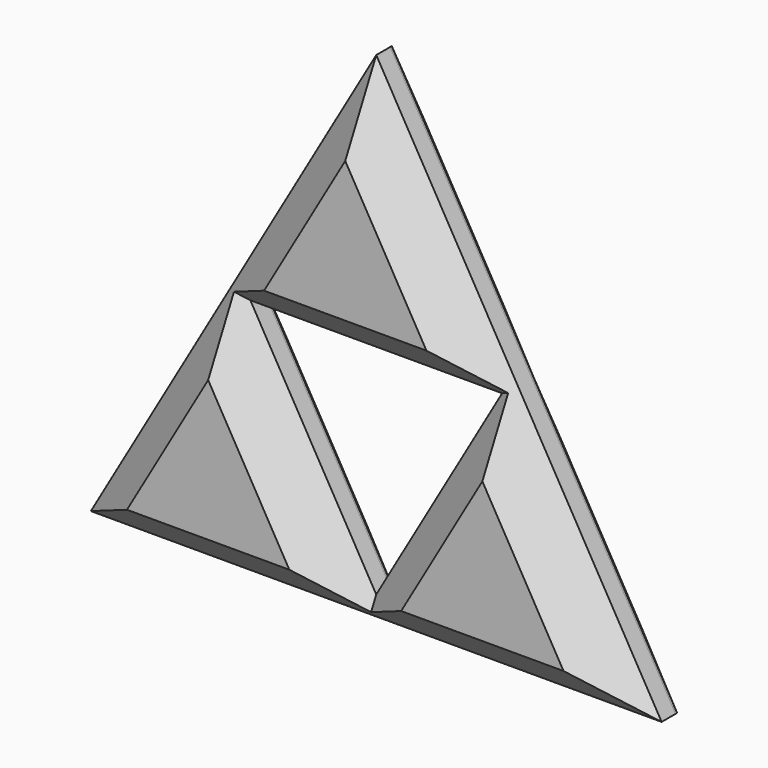
from build123d import *

# Parameters (mm, degrees)
F1_DEPTH      = 12.7
F2_T1_DEPTH   = 100.9671172602
F2_T3_DEPTH   = 100.9671172602
F2_T5_DEPTH   = 100.9671172602
F2_T10_DEPTH  = 59.1482991577
F2_T16_DEPTH  = 59.1482991577
F2_T22_DEPTH  = 59.1482991577
F2_T28_DEPTH  = 59.1482991577
F2_T34_DEPTH  = 59.1482991577
F2_T40_DEPTH  = 59.1482991577
F2_T47_DEPTH  = 59.1482991577
F2_T52_DEPTH  = 59.1482991577
F2_T60_DEPTH  = 59.1482991577
F2_T65_DEPTH  = 59.1482991577
F2_T73_DEPTH  = 59.1482991577
F2_T78_DEPTH  = 59.1482991577
F2_T86_DEPTH  = 59.1482991577
F2_T91_DEPTH  = 59.1482991577
F2_T99_DEPTH  = 59.1482991577
F2_T104_DEPTH = 59.1482991577
F2_T112_DEPTH = 59.1482991577
F2_T117_DEPTH = 59.1482991577
F3_DEPTH      = 2.286
F4_DEPTH      = 2.286


# Not quite as in the source:
# - a fillet or chamfer that OpenCascade refuses, or shapes differently, is made with other operations: its cross-section is extruded or revolved along the edge and cut away or added


with BuildPart() as f1:
    # F0 (on Front) → F1 (new body)
    with BuildSketch(Plane.XZ):
        Polygon((0, 57.1923176659), (-16.51, 28.596158833), (16.51, 28.596158833), align=None)
        Polygon((-33.02, 0), (0, 0), (-16.51, 28.596158833), align=None)
        Polygon((16.51, 28.596158833), (0, 0), (33.02, 0), align=None)
        Polygon((-37.4194090512, -2.54), (-33.02, 0), (-16.51, 28.596158833), (0, 57.1923176659), (0, 62.2723176659), align=None)
        Polygon((16.51, 28.596158833), (33.02, 0), (37.4194090512, -2.54), (0, 62.2723176659), (0, 57.1923176659), align=None)
        Polygon((33.02, 0), (0, 0), (-33.02, 0), (-37.4194090512, -2.54), (37.4194090512, -2.54), align=None)
    extrude(amount=F1_DEPTH)

    # F2: chamfer of 5.08 on 12 edges, made by hand

    # F2_s2 → F2_t1 (cut)
    with BuildSketch(Plane(origin=(33.496779315, 0, 58.0181236636), x_dir=(0, 1, 0), z_dir=(-0.5, 0, -0.8660254038))):
        Polygon((-7.62, -31.136158833), (-12.7, -26.056158833), (-12.7, -31.136158833), align=None)
        Polygon((-5.08, -31.136158833), (0, -26.056158833), (0, -31.136158833), align=None)
    extrude(amount=F2_T1_DEPTH, mode=Mode.SUBTRACT)

    # F2_s4 → F2_t3 (cut)
    with BuildSketch(Plane(origin=(16.986779315, 0, -29.4219648306), x_dir=(0, 1, 0), z_dir=(-0.5, 0, 0.8660254038))):
        Polygon((-7.62, -31.136158833), (-12.7, -26.056158833), (-12.7, -31.136158833), align=None)
        Polygon((-5.08, -31.136158833), (0, -26.056158833), (0, -31.136158833), align=None)
    extrude(amount=F2_T3_DEPTH, mode=Mode.SUBTRACT)

    # F2_s6 → F2_t5 (cut)
    with BuildSketch(Plane.YZ.offset(-50.4835586301)):
        Polygon((-7.62, -2.54), (-12.7, 2.54), (-12.7, -2.54), align=None)
        Polygon((-5.08, -2.54), (0, 2.54), (0, -2.54), align=None)
    extrude(amount=F2_T5_DEPTH, mode=Mode.SUBTRACT)


with BuildPart() as f2_tool8:
    # F2_s9 → F2_t10 (new body)
    with BuildSketch(Plane(origin=(6.5320747894, 0, -11.3138854141), x_dir=(0, 1, 0), z_dir=(-0.5, 0, 0.8660254038))):
        Polygon((-7.62, 0), (-12.7, 5.08), (-12.7, 0), align=None)
    extrude(amount=F2_T10_DEPTH)

    split(bisect_by=Plane(origin=(0, 0, 0), x_dir=(0, 1, 0), z_dir=(-0.8660254038, 0, 0.5)), keep=Keep.TOP)

    split(bisect_by=Plane.XY.offset(28.596158833), keep=Keep.BOTTOM)


with BuildPart() as f1_1:
    add(f1.part)

    # F2_t7: cut F2_tool8
    add(f2_tool8.part, mode=Mode.SUBTRACT)


with BuildPart() as f2_tool14:
    # F2_s15 → F2_t16 (new body)
    with BuildSketch(Plane.YZ.offset(-29.5741495789)):
        Polygon((-7.62, 28.596158833), (-12.7, 33.676158833), (-12.7, 28.596158833), align=None)
    extrude(amount=F2_T16_DEPTH)

    split(bisect_by=Plane(origin=(0, 0, 0), x_dir=(0, 1, 0), z_dir=(-0.8660254038, 0, 0.5)), keep=Keep.TOP)

    split(bisect_by=Plane(origin=(0, 0, 0), x_dir=(0, 1, 0), z_dir=(0.8660254038, 0, 0.5)), keep=Keep.TOP)


with BuildPart() as f1_2:
    add(f1_1.part)

    # F2_t13: cut F2_tool14
    add(f2_tool14.part, mode=Mode.SUBTRACT)


with BuildPart() as f2_tool20:
    # F2_s21 → F2_t22 (new body)
    with BuildSketch(Plane(origin=(23.0420747894, 0, 39.9100442471), x_dir=(0, 1, 0), z_dir=(-0.5, 0, -0.8660254038))):
        Polygon((-7.62, 0), (-12.7, 5.08), (-12.7, 0), align=None)
    extrude(amount=F2_T22_DEPTH)

    split(bisect_by=Plane(origin=(0, 0, 0), x_dir=(0, 1, 0), z_dir=(0.8660254038, 0, 0.5)), keep=Keep.TOP)

    split(bisect_by=Plane.XY.offset(28.596158833), keep=Keep.BOTTOM)


with BuildPart() as f1_3:
    add(f1_2.part)

    # F2_t19: cut F2_tool20
    add(f2_tool20.part, mode=Mode.SUBTRACT)


with BuildPart() as f2_tool26:
    # F2_s27 → F2_t28 (new body)
    with BuildSketch(Plane(origin=(23.0420747894, 0, 39.9100442471), x_dir=(0, 1, 0), z_dir=(-0.5, 0, -0.8660254038))):
        Polygon((-5.08, 0), (0, 5.08), (0, 0), align=None)
    extrude(amount=F2_T28_DEPTH)

    split(bisect_by=Plane(origin=(0, 0, 0), x_dir=(0, 1, 0), z_dir=(0.8660254038, 0, 0.5)), keep=Keep.TOP)

    split(bisect_by=Plane.XY.offset(28.596158833), keep=Keep.BOTTOM)


with BuildPart() as f1_4:
    add(f1_3.part)

    # F2_t25: cut F2_tool26
    add(f2_tool26.part, mode=Mode.SUBTRACT)


with BuildPart() as f2_tool32:
    # F2_s33 → F2_t34 (new body)
    with BuildSketch(Plane.YZ.offset(-29.5741495789)):
        Polygon((-5.08, 28.596158833), (0, 33.676158833), (0, 28.596158833), align=None)
    extrude(amount=F2_T34_DEPTH)

    split(bisect_by=Plane(origin=(0, 0, 0), x_dir=(0, 1, 0), z_dir=(-0.8660254038, 0, 0.5)), keep=Keep.TOP)

    split(bisect_by=Plane(origin=(0, 0, 0), x_dir=(0, 1, 0), z_dir=(0.8660254038, 0, 0.5)), keep=Keep.TOP)


with BuildPart() as f1_5:
    add(f1_4.part)

    # F2_t31: cut F2_tool32
    add(f2_tool32.part, mode=Mode.SUBTRACT)


with BuildPart() as f2_tool38:
    # F2_s39 → F2_t40 (new body)
    with BuildSketch(Plane(origin=(6.5320747894, 0, -11.3138854141), x_dir=(0, 1, 0), z_dir=(-0.5, 0, 0.8660254038))):
        Polygon((-5.08, 0), (0, 5.08), (0, 0), align=None)
    extrude(amount=F2_T40_DEPTH)

    split(bisect_by=Plane(origin=(0, 0, 0), x_dir=(0, 1, 0), z_dir=(-0.8660254038, 0, 0.5)), keep=Keep.TOP)

    split(bisect_by=Plane.XY.offset(28.596158833), keep=Keep.BOTTOM)


with BuildPart() as f1_6:
    add(f1_5.part)

    # F2_t37: cut F2_tool38
    add(f2_tool38.part, mode=Mode.SUBTRACT)


with BuildPart() as f2_tool45:
    # F2_s46 → F2_t47 (new body)
    with BuildSketch(Plane(origin=(23.0420747894, 0, 39.9100442471), x_dir=(0, 1, 0), z_dir=(-0.5, 0, -0.8660254038))):
        Polygon((-7.62, 0), (-12.7, 5.08), (-12.7, 0), align=None)
    extrude(amount=F2_T47_DEPTH)

    split(bisect_by=Plane.XY.offset(-2.54), keep=Keep.TOP)

    split(bisect_by=Plane(origin=(0, 0, 0), x_dir=(0, 1, 0), z_dir=(-0.8660254038, 0, -0.5)), keep=Keep.TOP)


with BuildPart() as f2_tool50:
    # F2_s51 → F2_t52 (new body)
    with BuildSketch(Plane(origin=(6.5320747894, 0, -11.3138854141), x_dir=(0, 1, 0), z_dir=(-0.5, 0, 0.8660254038))):
        Polygon((-7.62, 0), (-12.7, 5.08), (-12.7, 0), align=None)
    extrude(amount=F2_T52_DEPTH)

    split(bisect_by=Plane.XY.offset(-2.54), keep=Keep.TOP)

    split(bisect_by=Plane(origin=(0, 0, 0), x_dir=(0, 1, 0), z_dir=(0.8660254038, 0, -0.5)), keep=Keep.TOP)


with BuildPart() as f2_tool45_1:
    add(f2_tool45.part)

    # F2_t55: intersect F2_tool50
    add(f2_tool50.part, mode=Mode.INTERSECT)


with BuildPart() as f1_7:
    add(f1_6.part)

    # F2_t43: cut F2_tool45
    add(f2_tool45_1.part, mode=Mode.SUBTRACT)


with BuildPart() as f2_tool58:
    # F2_s59 → F2_t60 (new body)
    with BuildSketch(Plane(origin=(6.5320747894, 0, -11.3138854141), x_dir=(0, 1, 0), z_dir=(-0.5, 0, 0.8660254038))):
        Polygon((-7.62, 0), (-12.7, 5.08), (-12.7, 0), align=None)
    extrude(amount=F2_T60_DEPTH)

    split(bisect_by=Plane(origin=(-26.9647045256, 0, 15.5680794165), x_dir=(0, 1, 0), z_dir=(0.8660254038, 0, -0.5)), keep=Keep.TOP)

    split(bisect_by=Plane.XY.offset(28.596158833), keep=Keep.TOP)


with BuildPart() as f2_tool63:
    # F2_s64 → F2_t65 (new body)
    with BuildSketch(Plane.YZ.offset(-29.5741495789)):
        Polygon((-7.62, 28.596158833), (-12.7, 33.676158833), (-12.7, 28.596158833), align=None)
    extrude(amount=F2_T65_DEPTH)

    split(bisect_by=Plane(origin=(-26.9647045256, 0, 15.5680794165), x_dir=(0, 1, 0), z_dir=(0.8660254038, 0, -0.5)), keep=Keep.TOP)

    split(bisect_by=Plane(origin=(0, 0, 0), x_dir=(0, 1, 0), z_dir=(-0.8660254038, 0, -0.5)), keep=Keep.TOP)


with BuildPart() as f2_tool58_1:
    add(f2_tool58.part)

    # F2_t68: intersect F2_tool63
    add(f2_tool63.part, mode=Mode.INTERSECT)


with BuildPart() as f1_8:
    add(f1_7.part)

    # F2_t56: cut F2_tool58
    add(f2_tool58_1.part, mode=Mode.SUBTRACT)


with BuildPart() as f2_tool71:
    # F2_s72 → F2_t73 (new body)
    with BuildSketch(Plane(origin=(23.0420747894, 0, 39.9100442471), x_dir=(0, 1, 0), z_dir=(-0.5, 0, -0.8660254038))):
        Polygon((-7.62, 0), (-12.7, 5.08), (-12.7, 0), align=None)
    extrude(amount=F2_T73_DEPTH)

    split(bisect_by=Plane(origin=(26.9647045256, 0, 15.5680794165), x_dir=(0, 1, 0), z_dir=(-0.8660254038, 0, -0.5)), keep=Keep.TOP)

    split(bisect_by=Plane.XY.offset(28.596158833), keep=Keep.TOP)


with BuildPart() as f2_tool76:
    # F2_s77 → F2_t78 (new body)
    with BuildSketch(Plane.YZ.offset(-29.5741495789)):
        Polygon((-7.62, 28.596158833), (-12.7, 33.676158833), (-12.7, 28.596158833), align=None)
    extrude(amount=F2_T78_DEPTH)

    split(bisect_by=Plane(origin=(26.9647045256, 0, 15.5680794165), x_dir=(0, 1, 0), z_dir=(-0.8660254038, 0, -0.5)), keep=Keep.TOP)

    split(bisect_by=Plane(origin=(0, 0, 0), x_dir=(0, 1, 0), z_dir=(0.8660254038, 0, -0.5)), keep=Keep.TOP)


with BuildPart() as f2_tool71_1:
    add(f2_tool71.part)

    # F2_t81: intersect F2_tool76
    add(f2_tool76.part, mode=Mode.INTERSECT)


with BuildPart() as f1_9:
    add(f1_8.part)

    # F2_t69: cut F2_tool71
    add(f2_tool71_1.part, mode=Mode.SUBTRACT)


with BuildPart() as f2_tool84:
    # F2_s85 → F2_t86 (new body)
    with BuildSketch(Plane(origin=(23.0420747894, 0, 39.9100442471), x_dir=(0, 1, 0), z_dir=(-0.5, 0, -0.8660254038))):
        Polygon((-5.08, 0), (0, 5.08), (0, 0), align=None)
    extrude(amount=F2_T86_DEPTH)

    split(bisect_by=Plane(origin=(26.9647045256, 0, 15.5680794165), x_dir=(0, 1, 0), z_dir=(-0.8660254038, 0, -0.5)), keep=Keep.TOP)

    split(bisect_by=Plane.XY.offset(28.596158833), keep=Keep.TOP)


with BuildPart() as f2_tool89:
    # F2_s90 → F2_t91 (new body)
    with BuildSketch(Plane.YZ.offset(-29.5741495789)):
        Polygon((-5.08, 28.596158833), (0, 33.676158833), (0, 28.596158833), align=None)
    extrude(amount=F2_T91_DEPTH)

    split(bisect_by=Plane(origin=(26.9647045256, 0, 15.5680794165), x_dir=(0, 1, 0), z_dir=(-0.8660254038, 0, -0.5)), keep=Keep.TOP)

    split(bisect_by=Plane(origin=(0, 0, 0), x_dir=(0, 1, 0), z_dir=(0.8660254038, 0, -0.5)), keep=Keep.TOP)


with BuildPart() as f2_tool84_1:
    add(f2_tool84.part)

    # F2_t94: intersect F2_tool89
    add(f2_tool89.part, mode=Mode.INTERSECT)


with BuildPart() as f1_10:
    add(f1_9.part)

    # F2_t82: cut F2_tool84
    add(f2_tool84_1.part, mode=Mode.SUBTRACT)


with BuildPart() as f2_tool97:
    # F2_s98 → F2_t99 (new body)
    with BuildSketch(Plane(origin=(23.0420747894, 0, 39.9100442471), x_dir=(0, 1, 0), z_dir=(-0.5, 0, -0.8660254038))):
        Polygon((-5.08, 0), (0, 5.08), (0, 0), align=None)
    extrude(amount=F2_T99_DEPTH)

    split(bisect_by=Plane.XY.offset(-2.54), keep=Keep.TOP)

    split(bisect_by=Plane(origin=(0, 0, 0), x_dir=(0, 1, 0), z_dir=(-0.8660254038, 0, -0.5)), keep=Keep.TOP)


with BuildPart() as f2_tool102:
    # F2_s103 → F2_t104 (new body)
    with BuildSketch(Plane(origin=(6.5320747894, 0, -11.3138854141), x_dir=(0, 1, 0), z_dir=(-0.5, 0, 0.8660254038))):
        Polygon((-5.08, 0), (0, 5.08), (0, 0), align=None)
    extrude(amount=F2_T104_DEPTH)

    split(bisect_by=Plane.XY.offset(-2.54), keep=Keep.TOP)

    split(bisect_by=Plane(origin=(0, 0, 0), x_dir=(0, 1, 0), z_dir=(0.8660254038, 0, -0.5)), keep=Keep.TOP)


with BuildPart() as f2_tool97_1:
    add(f2_tool97.part)

    # F2_t107: intersect F2_tool102
    add(f2_tool102.part, mode=Mode.INTERSECT)


with BuildPart() as f1_11:
    add(f1_10.part)

    # F2_t95: cut F2_tool97
    add(f2_tool97_1.part, mode=Mode.SUBTRACT)


with BuildPart() as f2_tool110:
    # F2_s111 → F2_t112 (new body)
    with BuildSketch(Plane(origin=(6.5320747894, 0, -11.3138854141), x_dir=(0, 1, 0), z_dir=(-0.5, 0, 0.8660254038))):
        Polygon((-5.08, 0), (0, 5.08), (0, 0), align=None)
    extrude(amount=F2_T112_DEPTH)

    split(bisect_by=Plane(origin=(-26.9647045256, 0, 15.5680794165), x_dir=(0, 1, 0), z_dir=(0.8660254038, 0, -0.5)), keep=Keep.TOP)

    split(bisect_by=Plane.XY.offset(28.596158833), keep=Keep.TOP)


with BuildPart() as f2_tool115:
    # F2_s116 → F2_t117 (new body)
    with BuildSketch(Plane.YZ.offset(-29.5741495789)):
        Polygon((-5.08, 28.596158833), (0, 33.676158833), (0, 28.596158833), align=None)
    extrude(amount=F2_T117_DEPTH)

    split(bisect_by=Plane(origin=(-26.9647045256, 0, 15.5680794165), x_dir=(0, 1, 0), z_dir=(0.8660254038, 0, -0.5)), keep=Keep.TOP)

    split(bisect_by=Plane(origin=(0, 0, 0), x_dir=(0, 1, 0), z_dir=(-0.8660254038, 0, -0.5)), keep=Keep.TOP)


with BuildPart() as f2_tool110_1:
    add(f2_tool110.part)

    # F2_t120: intersect F2_tool115
    add(f2_tool115.part, mode=Mode.INTERSECT)


with BuildPart() as f1_12:
    add(f1_11.part)

    # F2_t108: cut F2_tool110
    add(f2_tool110_1.part, mode=Mode.SUBTRACT)

    # F3 (cut): faces of the model
    f3_faces = [f1_12.faces().sort_by_distance(p)[0] for p in [
        (-17.9764696838, -12.7, 8.6853862777),
        (-10.2690242997, -9.9455949432, 13.1352819449),
        (0, -9.9455949432, 30.9217537762),
        (-17.9764696838, -12.7, 8.6853862777),
        (10.2690242997, -9.9455949432, 13.1352819449),
        (-17.9764696838, -12.7, 8.6853862777),
        (10.2690242997, -9.9455949432, 13.1352819449),
        (23.7578772071, -12.1695918979, 12.0232834675),
        (-10.2690242997, -9.9455949432, 13.1352819449),
    ]]
    extrude(f3_faces, amount=-F3_DEPTH, dir=(0, -1, 0), mode=Mode.SUBTRACT)

    # F4 (add): faces of the model
    f4_faces = [f1_12.faces().sort_by_distance(p)[0] for p in [
        (-17.9764696838, -10.414, 8.6853862777),
        (-17.9764696838, -10.414, 8.6853862777),
        (-10.2690242997, -7.6595949432, 13.1352819449),
        (-17.9764696838, -10.414, 8.6853862777),
        (10.2690242997, -7.6595949432, 13.1352819449),
        (-10.2690242997, -7.6595949432, 13.1352819449),
        (0, -7.6595949432, 30.9217537762),
        (10.2690242997, -7.6595949432, 13.1352819449),
        (23.7578772071, -9.8835918979, 12.0232834675),
    ]]
    extrude(f4_faces, amount=F4_DEPTH, dir=(0, -1, 0))


solid = f1_12.part
